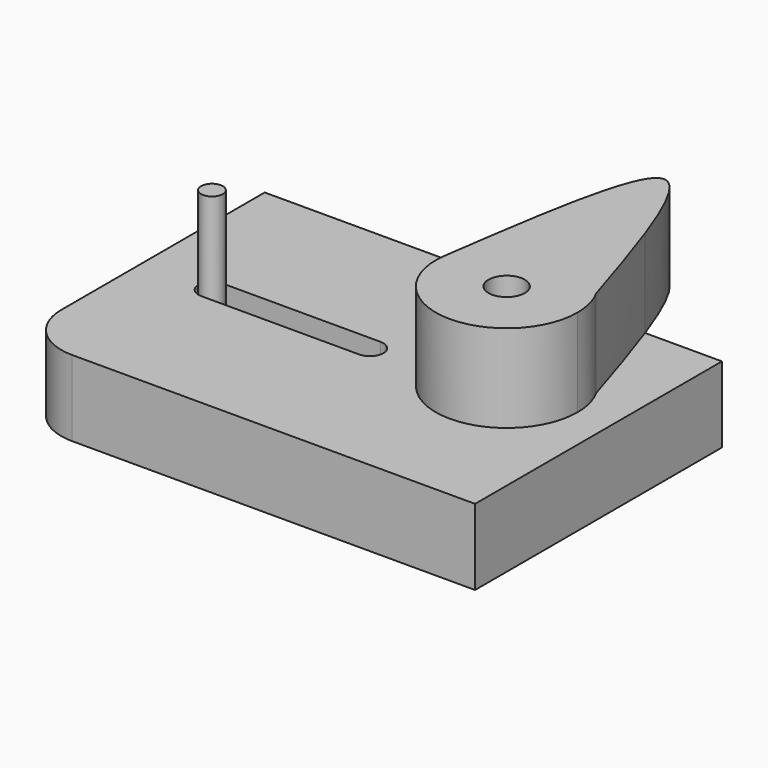
from build123d import *

# Parameters (mm, degrees)
F0_W          = 214.3064960837
F0_H          = 144.6259766817
F0_R          = 8.5081273079
F1_DEPTH      = 35.56
F3_R          = 5.08
F4_DEPTH      = 41.148
F4_DEPTH_BACK = 35.56
F2_R          = 8.5081273079
F5_DEPTH      = 41.148
F6_R          = 25.4


with BuildPart() as f1:
    # F0 (on Top) → F1 (new body)
    with BuildSketch(Plane.XY):
        with Locations((-142.4723118544, 46.1902879179)):
            Rectangle(F0_W, F0_H)
        with BuildLine():
            Line((-142.4723118544, 39.8402879179), (-216.4897322655, 39.8402879179))
            ThreePointArc((-216.4897322655, 39.8402879179), (-222.8397322655, 46.1902879179), (-216.4897322655, 52.5402879179))
            Line((-216.4897322655, 52.5402879179), (-142.4723118544, 52.5402879179))
            ThreePointArc((-142.4723118544, 52.5402879179), (-136.1223118544, 46.1902879179), (-142.4723118544, 39.8402879179))
        make_face(mode=Mode.SUBTRACT)
        with Locations((-84.6008360386, 53.9804883301)):
            Circle(F0_R, mode=Mode.SUBTRACT)
    extrude(amount=F1_DEPTH)

    # F6
    f6_edges = [f1.edges().sort_by_distance(p)[0] for p in [
        (-249.62556, -26.1227, 17.78),
    ]]
    fillet(f6_edges, radius=F6_R)


with BuildPart() as f4:
    # F3 (on face) → F4 (new body, two sides)
    with BuildSketch(Plane.XY.offset(35.56)) as f4_sk:
        with Locations((-216.4897322655, 46.1902879179)):
            Circle(F3_R)
    extrude(amount=F4_DEPTH)
    extrude(f4_sk.sketch, amount=-F4_DEPTH_BACK)


with BuildPart() as f5:
    # F2 (on face) → F5 (new body, through all)
    with BuildSketch(Plane.XY.offset(35.56)):
        with BuildLine():
            ThreePointArc((-117.4909419259, 58.6982221516), (-86.9657003677, 20.8380156645), (-51.374098647, 53.9804883301))
            ThreePointArc((-51.374098647, 53.9804883301), (-52.4269300084, 62.2784307525), (-55.5187034955, 70.0505114923))
            ThreePointArc((-55.5187034955, 70.0505114923), (-90.5878038493, 86.6633935578), (-117.4909419259, 58.6982221516))
        make_face()
        with Locations((-84.6008360386, 53.9804883301)):
            Circle(F2_R, mode=Mode.SUBTRACT)
        with BuildLine():
            ThreePointArc((-117.4909419259, 58.6982221516), (-90.5878038493, 86.6633935578), (-55.5187034955, 70.0505114923))
            add(Edge.make_bspline(
                [(-71.3437874184, 118.5032762587), (-66.2032422505, 104.1232170214), (-60.8587807347, 87.0871227133), (-55.5187034955, 70.0505114923)],
                knots=[0.8077687056, 0.8077687056, 0.8077687056, 0.8077687056, 1, 1, 1, 1], degree=3))
            Line((-71.3437874184, 118.5032762587), (-108.0454849884, 118.5032762587))
            add(Edge.make_bspline(
                [(-117.4909419259, 58.6982221516), (-114.4385454829, 79.97827864), (-111.3965044358, 101.2627998667), (-108.0454849884, 118.5032762587)],
                knots=[0, 0, 0, 0, 0.2236901556, 0.2236901556, 0.2236901556, 0.2236901556], degree=3))
        make_face()
        with BuildLine():
            Line((-108.0454849884, 118.5032762587), (-71.3437874184, 118.5032762587))
            add(Edge.make_bspline(
                [(-108.0454849884, 118.5032762587), (-103.7805881801, 140.4455102242), (-94.0039277475, 172.0230555596), (-79.3497645207, 140.8990380359), (-71.3437874184, 118.5032762587)],
                knots=[0.2236901556, 0.2236901556, 0.2236901556, 0.2236901556, 0.5083842451, 0.8077687056, 0.8077687056, 0.8077687056, 0.8077687056], degree=3))
        make_face()
    extrude(amount=F5_DEPTH)


solid = Compound([f1.part, f4.part, f5.part])
